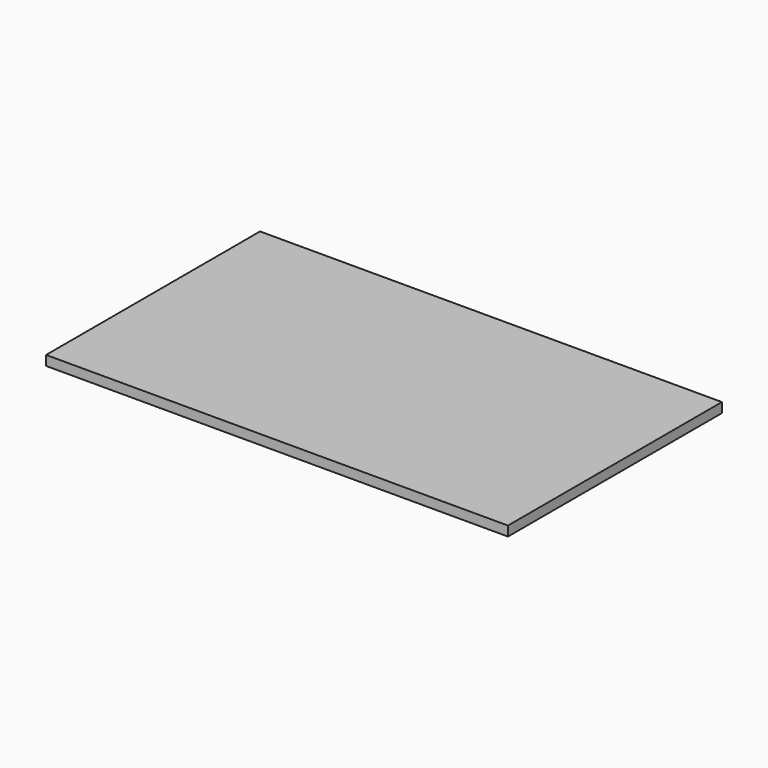
from build123d import *

# Parameters (mm, degrees)
F0_W     = 95
F0_H     = 55
F1_DEPTH = 2


# Not quite as in the source:
# - a feature names something its author has since deleted; it is built from what else it names


with BuildPart() as f1:
    # F0 (on Top) → F1 (new body)
    with BuildSketch(Plane.XY):
        with Locations((17.6483844221, -5.0764417648)):
            Rectangle(F0_W, F0_H)
    extrude(amount=F1_DEPTH)


solid = f1.part
